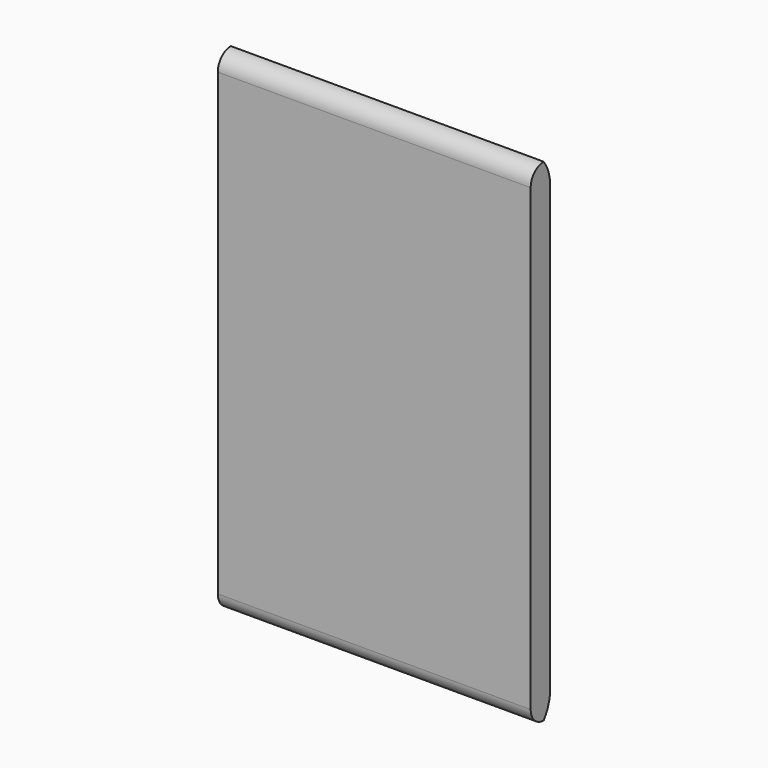
from build123d import *

# Parameters (mm, degrees)
F3_DEPTH     = 7.62
F4_DEPTH     = 4.318
F1_W         = 86.36
F1_H         = 55.88
F5_DEPTH     = 3.81
F6_W         = 6.2699629925
F6_H         = 43.1555788964
F7_DEPTH     = 4.572
F8_R         = 5.08
F9_T1_DEPTH  = 135.8469622158
F10_R        = 5.08
F11_T1_DEPTH = 135.8469622158


# Not quite as in the source:
# - a fillet or chamfer that OpenCascade refuses, or shapes differently, is made with other operations: its cross-section is extruded or revolved along the edge and cut away or added


with BuildPart() as f3:
    # F2 (on Front) → F3 (new body)
    with BuildSketch(Plane.XZ):
        Polygon((-6.2699629925, 72.1773862183), (-6.2699629925, 59.4773862183), (-6.2699629925, -68.8154984593), (-6.2699629925, -81.5154984593), (91.4769992232, -81.5154984593), (91.4769992232, -68.8154984593), (91.4769992232, 59.4773862183), (91.4769992232, 72.1773862183), align=None)
    extrude(amount=F3_DEPTH)

    # F0 (on Front) → F4 (cut)
    with BuildSketch(Plane.XZ):
        Polygon((0, 53.34), (0, 0), (66.5871798992, 0), (70.5303996801, 0), (78.1503996801, 0), (78.1503996801, 53.34), (70.5303996801, 53.34), (64.516, 53.34), align=None)
    extrude(amount=F4_DEPTH, mode=Mode.SUBTRACT)

    # F1 (on Front) → F5 (cut)
    with BuildSketch(Plane.XZ):
        with Locations((43.18, -36.3771444535)):
            Rectangle(F1_W, F1_H)
    extrude(amount=F5_DEPTH, mode=Mode.SUBTRACT)

    # F6 (on face) → F7 (cut)
    with BuildSketch(Plane(origin=(0, 0, 0), x_dir=(-1, 0, 0), z_dir=(0, 1, 0))):
        with Locations((3.1349814963, 28.3439913765)):
            Rectangle(F6_W, F6_H)
    extrude(amount=-F7_DEPTH, mode=Mode.SUBTRACT)

    # F8
    f8_edges = [f3.edges().sort_by_distance(p)[0] for p in [
        (42.603518, -7.62, -81.515498),
    ]]
    fillet(f8_edges, radius=F8_R)

    # F9: fillet of radius 12.7 on 1 edges, made by hand

    # F9_s2 → F9_t1 (cut)
    with BuildSketch(Plane.YZ.offset(-25.3199629925)):
        with BuildLine():
            ThreePointArc((-2.54, -81.5154984593), (-0.6517221148, -77.9115910878), (0, -73.8954984593))
            Line((0, -73.8954984593), (0, -81.5154984593))
            Line((0, -81.5154984593), (-2.54, -81.5154984593))
        make_face()
    extrude(amount=F9_T1_DEPTH, mode=Mode.SUBTRACT)

    # F10
    f10_edges = [f3.edges().sort_by_distance(p)[0] for p in [
        (42.603518, -7.62, 72.177386),
    ]]
    fillet(f10_edges, radius=F10_R)

    # F11: fillet of radius 12.7 on 1 edges, made by hand

    # F11_s2 → F11_t1 (cut)
    with BuildSketch(Plane.YZ.offset(-25.3199629925)):
        with BuildLine():
            ThreePointArc((-2.54, 72.1773862183), (-0.6517221148, 68.5734788467), (0, 64.5573862183))
            Line((0, 64.5573862183), (0, 72.1773862183))
            Line((0, 72.1773862183), (-2.54, 72.1773862183))
        make_face()
    extrude(amount=F11_T1_DEPTH, mode=Mode.SUBTRACT)


solid = f3.part
